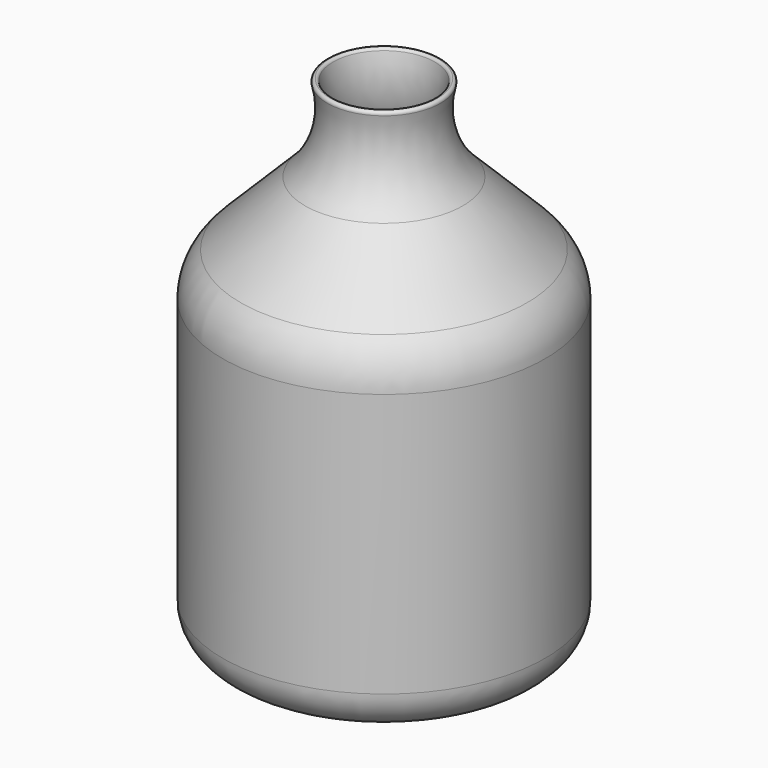
from build123d import *

# Parameters (mm, degrees)
F2_T = -5.08


# Not quite as in the source:
# - a fillet or chamfer that OpenCascade refuses, or shapes differently, is made with other operations: its cross-section is extruded or revolved along the edge and cut away or added


with BuildPart() as f1:
    # F0 (on Front) → F1 (revolve)
    with BuildSketch(Plane.XZ):
        with BuildLine():
            Line((-104.749092273, 0), (0, 0))
            Line((0, 0), (0, 431.8))
            Line((0, 431.8), (-49.921810742, 431.8))
            ThreePointArc((-49.921810742, 431.8), (-48.6708978442, 391.6994834486), (-68.3686659031, 356.7478862853))
            Line((-68.3686659031, 356.7478862853), (-124.1141319396, 301.0024202488))
            ThreePointArc((-124.1141319396, 301.0024202488), (-135.6493648648, 283.7387241792), (-139.7, 263.374806196))
            Line((-139.7, 263.374806196), (-139.7, 34.950907727))
            ThreePointArc((-139.7, 34.950907727), (-129.4631161354, 10.2368838646), (-104.749092273, 0))
        make_face()
    revolve(axis=Axis((0, 0, 215.9), (0, 0, -1)))

    # F2
    f2_openings = [f1.faces().sort_by_distance(p)[0] for p in [
        (0, 0, 431.8),
    ]]
    offset(amount=F2_T, openings=f2_openings)

    # F3: fillet of radius 2.54 on 2 edges, made by hand

    # F3_s1 → F3_t2 (revolve, cut)
    with BuildSketch(Plane.XZ):
        with BuildLine():
            ThreePointArc((-49.0005618222, 428.6097837881), (-48.558048849, 430.8092015398), (-46.5451964974, 431.8))
            Line((-46.5451964974, 431.8), (-49.921810742, 431.8))
            ThreePointArc((-49.921810742, 431.8), (-49.4434375246, 430.2100172594), (-49.0005618222, 428.6097837881))
        make_face()
    revolve(axis=Axis((0, 0, 431.8), (0, 0, -1)), mode=Mode.SUBTRACT)

    # F3_s3 → F3_t4 (revolve, cut)
    with BuildSketch(Plane.XZ):
        with BuildLine():
            ThreePointArc((-46.5451964974, 431.8), (-44.9959949577, 431.2728523515), (-44.0898311727, 429.9102162119))
            ThreePointArc((-44.0898311727, 429.9102162119), (-44.3467229528, 430.8567245972), (-44.6152430168, 431.8))
            Line((-44.6152430168, 431.8), (-46.5451964974, 431.8))
        make_face()
    revolve(axis=Axis((0, 0, 431.8), (0, 0, 1)), mode=Mode.SUBTRACT)


solid = f1.part
